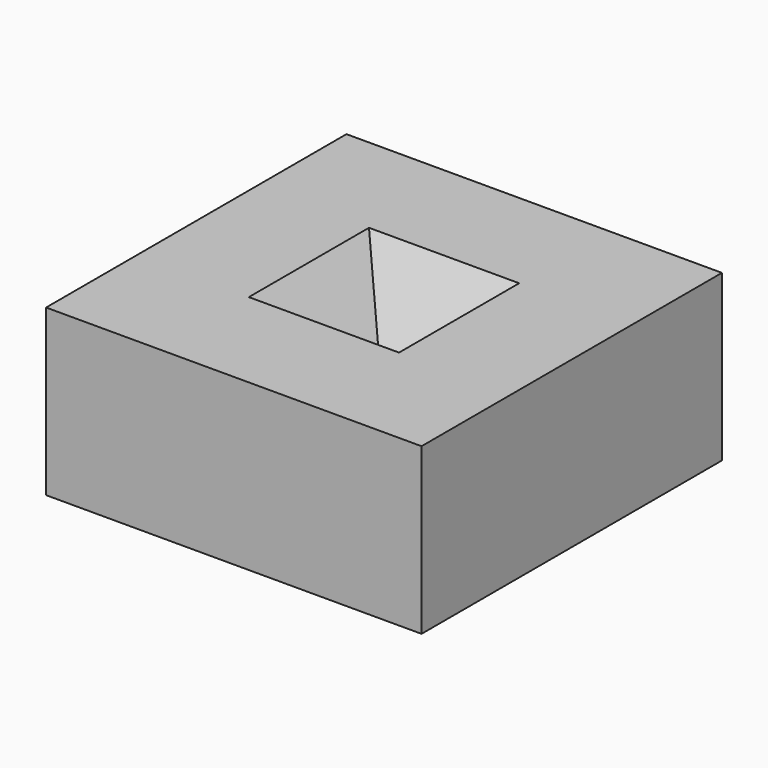
from build123d import *

# Parameters (mm, degrees)
F0_W     = 50
F0_H     = 50
F2_DEPTH = 22
F1_W     = 20
F1_H     = 20


# Not quite as in the source:
# - an extrude whose draft closes it to a point is written as a loft to that point


with BuildPart() as f2:
    # F0 (on Top) → F2 (new body)
    with BuildSketch(Plane.XY):
        Rectangle(F0_W, F0_H)
    extrude(amount=-F2_DEPTH)

    # F1 (on Top) → F3 section 0
    with BuildSketch(Plane.XY, mode=Mode.PRIVATE) as f3_s0:
        Rectangle(F1_W, F1_H)
    loft([f3_s0.sketch, Vertex(0, 0, -15.3986496381)], ruled=True, mode=Mode.SUBTRACT)


solid = f2.part
